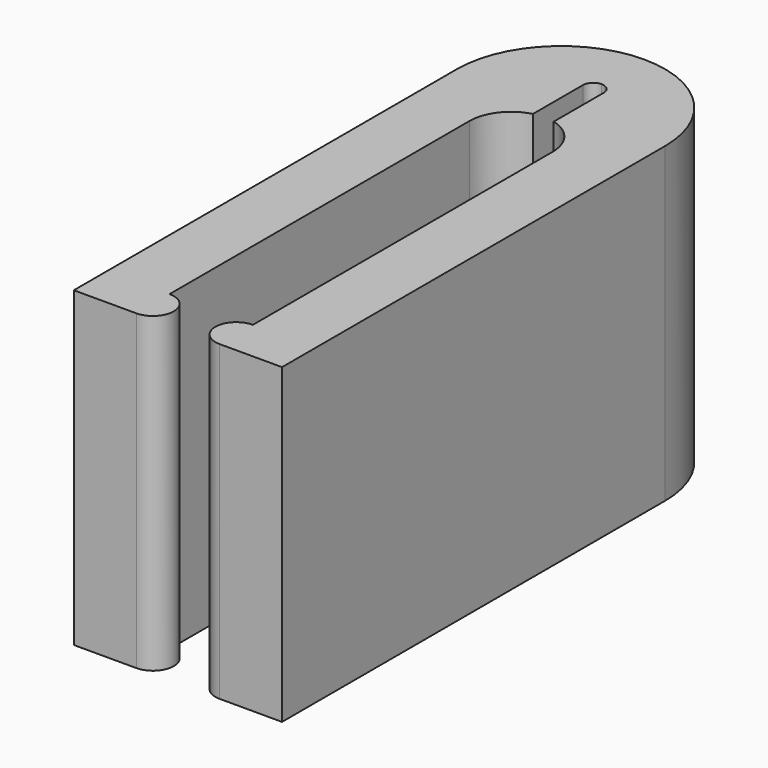
from build123d import *

# Parameters (mm, degrees)
F1_DEPTH = 15
F2_R     = 0.49999


# Not quite as in the source:
# - a fillet or chamfer is up to 0.001 mm smaller than in the source, because OpenCascade refuses the exact size


with BuildPart() as f1:
    # F0 (on Top) → F1 (new body)
    with BuildSketch(Plane.XY):
        with BuildLine():
            Line((-5, -12.237534521), (-2, -12.237534521))
            ThreePointArc((-2, -12.237534521), (-1, -11.237534521), (-2, -10.237534521))
            Line((-2, -10.237534521), (-2, 7.762465479))
            ThreePointArc((-2, 7.762465479), (-1.5811388301, 8.9872103504), (-0.5, 9.6989571521))
            Line((-0.5, 9.6989571521), (-0.5, 13.1989571521))
            Line((-0.5, 13.1989571521), (0.5, 13.1989571521))
            Line((0.5, 13.1989571521), (0.5, 9.6989571521))
            ThreePointArc((0.5, 9.6989571521), (1.5811388301, 8.9872103504), (2, 7.762465479))
            Line((2, 7.762465479), (2, -10.237534521))
            ThreePointArc((2, -10.237534521), (1, -11.237534521), (2, -12.237534521))
            Line((2, -12.237534521), (5, -12.237534521))
            Line((5, -12.237534521), (5, 10.762465479))
            ThreePointArc((5, 10.762465479), (0, 15.762465479), (-5, 10.762465479))
            Line((-5, 10.762465479), (-5, -12.237534521))
        make_face()
    extrude(amount=F1_DEPTH)

    # F2 (radius 0.5 in the source; OpenCascade refuses exactly that, so slightly less here)
    f2_edges = [f1.edges().sort_by_distance(p)[0] for p in [
        (-0.5, 13.198957, 7.5),
        (0.5, 13.198957, 7.5),
    ]]
    fillet(f2_edges, radius=F2_R)


solid = f1.part
